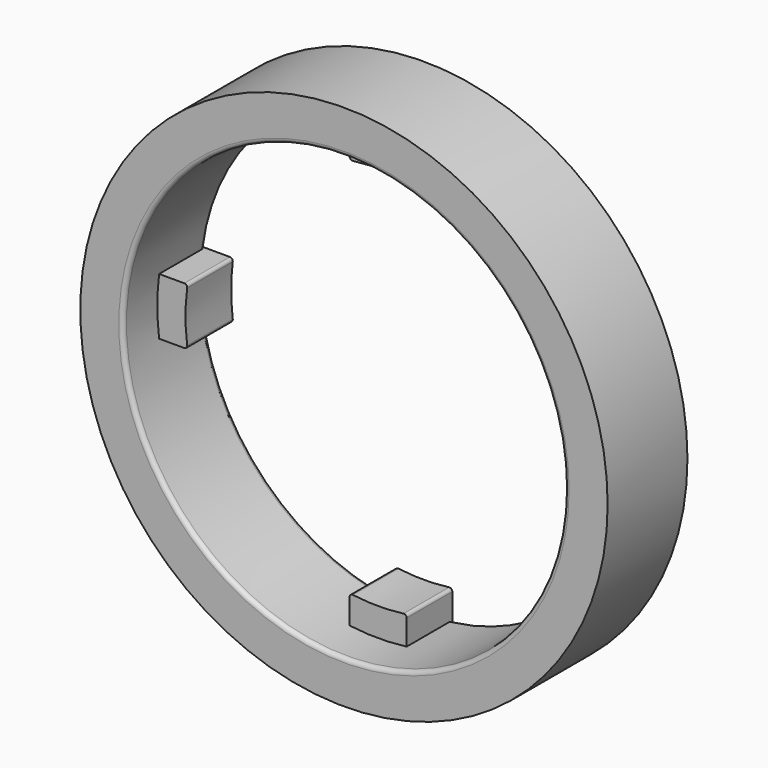
from build123d import *

# Parameters (mm, degrees)
F0_R            = 18.5
F0_R_2          = 15.5
F1_DEPTH        = 7
F3_DEPTH        = 4
F3_COPIES_COUNT = 4
F4_R            = 0.2
F5_T6_ANGLE     = 80.7189590371
F5_T12_ANGLE    = 80.7189590371
F5_T18_ANGLE    = 80.7189590371
F5_T24_ANGLE    = 80.7189590371


# Not quite as in the source:
# - a fillet or chamfer that OpenCascade refuses, or shapes differently, is made with other operations: its cross-section is extruded or revolved along the edge and cut away or added
# - a pattern or mirror of a feature is missing from the dataset's text; its kind, count and spacing are read off the source's solid


with BuildPart() as f1:
    # F0 (on Front) → F1 (new body)
    with BuildSketch(Plane.XZ):
        Circle(F0_R)
        Circle(F0_R_2, mode=Mode.SUBTRACT)
    extrude(amount=F1_DEPTH)

    # F2 (on Front) → F3 (join)
    with BuildSketch(Plane.XZ):
        with BuildLine():
            ThreePointArc((-2, 13.3704261489), (0, 13.5191824976), (2, 13.3704261489))
            Line((2, 13.3704261489), (2, 15.3704261489))
            ThreePointArc((2, 15.3704261489), (0, 15.5), (-2, 15.3704261489))
            Line((-2, 15.3704261489), (-2, 13.3704261489))
        make_face()
    f3 = extrude(amount=F3_DEPTH)

    # F3_copies: F3 ×4 about axis
    f3_copies_axis = Axis((0, 0, 0), (0, 1, 0))
    for i in range(1, F3_COPIES_COUNT):
        add(f3.rotate(f3_copies_axis, i * 360 / F3_COPIES_COUNT))

    # F4
    f4_edges = [f1.edges().sort_by_distance(p)[0] for p in [
        (2, -2, 13.370426),
        (-2, -2, 13.370426),
        (13.370426, -2, 2),
        (13.370426, -2, -2),
        (2, -2, -13.370426),
        (-2, -2, -13.370426),
        (-13.370426, -2, 2),
        (-13.370426, -2, -2),
    ]]
    fillet(f4_edges, radius=F4_R)

    # F5: fillet of radius 0.3 on 5 edges, made by hand

    # F5_s1 → F5_t2 (revolve, cut)
    with BuildSketch(Plane.XY):
        with BuildLine():
            ThreePointArc((15.5, -6.7), (15.5878679656, -6.9121320344), (15.8, -7))
            Line((15.8, -7), (15.5, -7))
            Line((15.5, -7), (15.5, -6.7))
        make_face()
    revolve(axis=Axis((0, -7, 0), (0, -1, 0)), mode=Mode.SUBTRACT)


with BuildPart() as f5_tool4:
    # F5_s5 → F5_t6 (revolve)
    with BuildSketch(Plane(origin=(0, 0, 0), x_dir=(0, 1, 0), z_dir=(0.080903842, 0, -0.9967219112))):
        with BuildLine():
            ThreePointArc((0, 15.8), (-0.0878679656, 15.5878679656), (-0.3, 15.5))
            Line((-0.3, 15.5), (0, 15.5))
            Line((0, 15.5), (0, 15.8))
        make_face()
    revolve(axis=Axis((0, 0, 0), (0, -1, 0)), revolution_arc=F5_T6_ANGLE)

    split(bisect_by=Plane.XY.offset(2), keep=Keep.TOP)

    split(bisect_by=Plane.YZ.offset(2), keep=Keep.TOP)


with BuildPart() as f1_1:
    add(f1.part)

    # F5_t3: cut F5_tool4
    add(f5_tool4.part, mode=Mode.SUBTRACT)


with BuildPart() as f5_tool10:
    # F5_s11 → F5_t12 (revolve)
    with BuildSketch(Plane(origin=(0, 0, 0), x_dir=(0, 1, 0), z_dir=(-0.9967219112, 0, -0.080903842))):
        with BuildLine():
            ThreePointArc((0, 15.8), (-0.0878679656, 15.5878679656), (-0.3, 15.5))
            Line((-0.3, 15.5), (0, 15.5))
            Line((0, 15.5), (0, 15.8))
        make_face()
    revolve(axis=Axis((0, 0, 0), (0, -1, 0)), revolution_arc=F5_T12_ANGLE)

    split(bisect_by=Plane.XY.offset(-2), keep=Keep.BOTTOM)

    split(bisect_by=Plane.YZ.offset(2), keep=Keep.TOP)


with BuildPart() as f1_2:
    add(f1_1.part)

    # F5_t9: cut F5_tool10
    add(f5_tool10.part, mode=Mode.SUBTRACT)


with BuildPart() as f5_tool16:
    # F5_s17 → F5_t18 (revolve)
    with BuildSketch(Plane(origin=(0, 0, 0), x_dir=(0, 1, 0), z_dir=(0.9967219112, 0, 0.080903842))):
        with BuildLine():
            ThreePointArc((0, 15.8), (-0.0878679656, 15.5878679656), (-0.3, 15.5))
            Line((-0.3, 15.5), (0, 15.5))
            Line((0, 15.5), (0, 15.8))
        make_face()
    revolve(axis=Axis((0, 0, 0), (0, -1, 0)), revolution_arc=F5_T18_ANGLE)

    split(bisect_by=Plane.YZ.offset(-2), keep=Keep.BOTTOM)

    split(bisect_by=Plane.XY.offset(2), keep=Keep.TOP)


with BuildPart() as f1_3:
    add(f1_2.part)

    # F5_t15: cut F5_tool16
    add(f5_tool16.part, mode=Mode.SUBTRACT)


with BuildPart() as f5_tool22:
    # F5_s23 → F5_t24 (revolve)
    with BuildSketch(Plane(origin=(0, 0, 0), x_dir=(0, 1, 0), z_dir=(-0.080903842, 0, 0.9967219112))):
        with BuildLine():
            ThreePointArc((0, 15.8), (-0.0878679656, 15.5878679656), (-0.3, 15.5))
            Line((-0.3, 15.5), (0, 15.5))
            Line((0, 15.5), (0, 15.8))
        make_face()
    revolve(axis=Axis((0, 0, 0), (0, -1, 0)), revolution_arc=F5_T24_ANGLE)

    split(bisect_by=Plane.YZ.offset(-2), keep=Keep.BOTTOM)

    split(bisect_by=Plane.XY.offset(-2), keep=Keep.BOTTOM)


with BuildPart() as f1_4:
    add(f1_3.part)

    # F5_t21: cut F5_tool22
    add(f5_tool22.part, mode=Mode.SUBTRACT)


solid = f1_4.part
